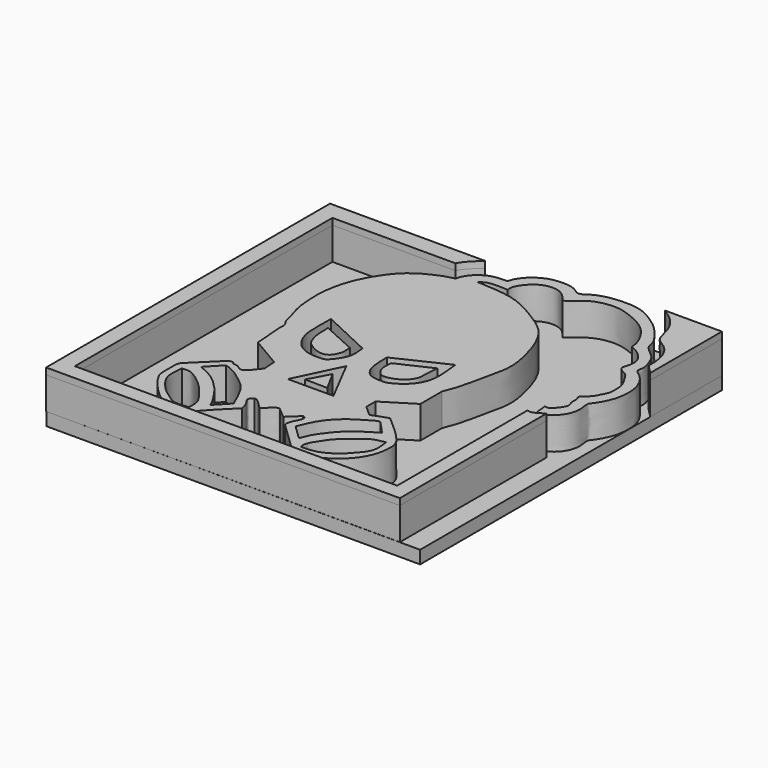
from build123d import *

# Parameters (mm, degrees)
F1_DEPTH = 5
F2_DEPTH = 1
F4_DEPTH = 2


# Not quite as in the source:
# - a feature names something its author has since deleted; it is built from what else it names


with BuildPart() as f1:
    # F0 (on Top) → F1 (new body)
    with BuildSketch(Plane.XY):
        with BuildLine():
            add(Edge.make_bspline(
                [(51.4540672302, 60.837585479), (51.9638869737, 60.5286784114), (53.1057350795, 59.8368163278), (54.9989821715, 57.6432839724), (55.3530510623, 54.4029967917), (56.8689093893, 53.8008966691), (58.5125441808, 52.2408419295), (59.0050335955, 49.7109659804), (58.9545683424, 48.7642556957), (58.9334107935, 48.3673475683)],
                knots=[0, 0, 0, 0, 0.1341689236, 0.3004994084, 0.4702111044, 0.5875997416, 0.7323290574, 0.8877790024, 1, 1, 1, 1], degree=3))
            add(Edge.make_bspline(
                [(58.9334107935, 48.3673475683), (59.3921567003, 47.8968396783), (59.850902607, 47.4263317883), (60.3096485138, 46.9558238983)],
                knots=[0, 0, 0, 0, 1.9714028846, 1.9714028846, 1.9714028846, 1.9714028846], degree=3))
            add(Edge.make_bspline(
                [(60.3096485138, 46.9558238983), (60.3096485138, 51.5830777586), (60.3096485138, 56.2103316188), (60.3096485138, 60.837585479)],
                knots=[0, 0, 0, 0, 13.8817615807, 13.8817615807, 13.8817615807, 13.8817615807], degree=3))
            add(Edge.make_bspline(
                [(60.3096485138, 60.837585479), (57.3577880859, 60.837585479), (54.4059276581, 60.837585479), (51.4540672302, 60.837585479)],
                knots=[0, 0, 0, 0, 8.8555812836, 8.8555812836, 8.8555812836, 8.8555812836], degree=3))
        make_face()
    extrude(amount=F1_DEPTH)


with BuildPart() as f1b:
    # F0 (on Top) → F1, piece 2 (new body)
    with BuildSketch(Plane.XY):
        with BuildLine():
            add(Edge.make_bspline(
                [(4.8520560376, 4.860504996), (21.518412667, 4.8331838722), (38.1847692964, 4.8058627484), (54.8511259258, 4.7785416245)],
                knots=[0, 0, 0, 0, 49.9991370693, 49.9991370693, 49.9991370693, 49.9991370693], degree=3))
            add(Edge.make_bspline(
                [(4.9181785434, 54.6599179506), (4.8961377082, 38.0601136324), (4.8740968729, 21.4603093142), (4.8520560376, 4.860504996)],
                knots=[0, 0, 0, 0, 49.7994568525, 49.7994568525, 49.7994568525, 49.7994568525], degree=3))
            add(Edge.make_bspline(
                [(23.9754598588, 54.6599179506), (17.6230327537, 54.6599179506), (11.2706056486, 54.6599179506), (4.9181785434, 54.6599179506)],
                knots=[0, 0, 0, 0, 19.0572813153, 19.0572813153, 19.0572813153, 19.0572813153], degree=3))
            add(Edge.make_bspline(
                [(26.3510439545, 57.3983192444), (25.3768845665, 56.4834475414), (24.4027251785, 55.5685758385), (23.9754598588, 54.6599179506)],
                knots=[0, 0, 0, 0, 0.5683118299, 0.5683118299, 0.5683118299, 0.5683118299], degree=3))
            add(Edge.make_bspline(
                [(2.3493634071, 57.3983192444), (10.5748367496, 57.3983192444), (18.125570612, 57.3983192444), (26.3510439545, 57.3983192444)],
                knots=[0, 0, 0, 0, 24.0016805474, 24.0016805474, 24.0016805474, 24.0016805474], degree=3))
            add(Edge.make_bspline(
                [(2.3493634071, 2.4174780119), (2.3493634071, 20.7312301112), (2.3493634071, 39.0845671451), (2.3493634071, 57.3983192444)],
                knots=[0, 0, 0, 0, 54.9808412325, 54.9808412325, 54.9808412325, 54.9808412325], degree=3))
            add(Edge.make_bspline(
                [(57.154417038, 2.4174780119), (38.8860658277, 2.4174780119), (20.6177146174, 2.4174780119), (2.3493634071, 2.4174780119)],
                knots=[0, 0, 0, 0, 54.8050536308, 54.8050536308, 54.8050536308, 54.8050536308], degree=3))
            add(Edge.make_bspline(
                [(57.154417038, 30.8391451836), (57.154417038, 21.3652561263), (57.154417038, 11.8913670691), (57.154417038, 2.4174780119)],
                knots=[0, 0, 0, 0, 28.4216671716, 28.4216671716, 28.4216671716, 28.4216671716], degree=3))
            add(Edge.make_bspline(
                [(56.1751872301, 30.2456729114), (56.3446747926, 30.3468590463), (56.7052673113, 30.5024971432), (57.0361231665, 30.7883044027), (57.154417038, 30.8391451836)],
                knots=[0.4614999783, 0.4614999783, 0.4614999783, 0.4614999783, 0.6787072438, 0.881944889, 0.881944889, 0.881944889, 0.881944889], degree=3))
            add(Edge.make_bspline(
                [(54.8511259258, 29.9786105752), (55.1455810804, 29.9474229205), (55.6857627215, 29.8902087804), (56.0113746232, 30.147874794), (56.1751872301, 30.2456729114)],
                knots=[0, 0, 0, 0, 0.2515654682, 0.4614999783, 0.4614999783, 0.4614999783, 0.4614999783], degree=3))
            add(Edge.make_bspline(
                [(54.8511259258, 29.7412201762), (54.8511259258, 29.8203503092), (54.8511259258, 29.8994804422), (54.8511259258, 29.9786105752)],
                knots=[0, 0, 0, 0, 0.237390399, 0.237390399, 0.237390399, 0.237390399], degree=3))
            add(Edge.make_bspline(
                [(54.8511259258, 4.7785416245), (54.8511259258, 13.0994344751), (54.8511259258, 21.4203273257), (54.8511259258, 29.7412201762)],
                knots=[0, 0, 0, 0, 24.9626785517, 24.9626785517, 24.9626785517, 24.9626785517], degree=3))
        make_face()
    extrude(amount=F1_DEPTH)


with BuildPart() as f1c:
    # F0 (on Top) → F1, piece 3 (new body)
    with BuildSketch(Plane.XY):
        with BuildLine():
            add(Edge.make_bspline(
                [(23.6329138279, 52.5964461267), (24.1818682601, 52.7461618185), (24.7308226923, 52.8958775103), (25.2797771245, 53.0455932021)],
                knots=[0, 0, 0, 0, 1.7070125404, 1.7070125404, 1.7070125404, 1.7070125404], degree=3))
            add(Edge.make_bspline(
                [(16.6953094304, 29.7442097217), (16.7411494158, 30.0597253678), (16.8346932753, 30.703585765), (16.1172664025, 31.527469058), (15.9920702036, 32.4892911415), (15.5262018988, 33.9022358039), (14.9877927895, 35.7559845442), (14.8019028777, 39.1876871759), (14.9425896683, 41.0184854519), (15.5349488179, 44.2279557805), (17.7090883866, 48.4871885716), (20.3947770421, 51.2022443546), (22.5699612299, 52.1387846708), (23.6329138279, 52.5964461267)],
                knots=[0, 0, 0, 0, 0.0581906098, 0.1187472939, 0.1778066529, 0.2499088208, 0.3358728435, 0.446880626, 0.5297458769, 0.6369929361, 0.7699468037, 0.8875793397, 1, 1, 1, 1], degree=3))
            add(Edge.make_bspline(
                [(16.6953094304, 29.7442097217), (16.8189499527, 28.1764511019), (16.9425904751, 26.6086924821), (17.0662309974, 25.0409338623)],
                knots=[0, 0, 0, 0, 4.717879462, 4.717879462, 4.717879462, 4.717879462], degree=3))
            add(Edge.make_bspline(
                [(17.0662309974, 25.0409338623), (18.6460409313, 24.1130304833), (20.2258508652, 23.1851271043), (21.8056607991, 22.2572237253)],
                knots=[0, 0, 0, 0, 5.4964749587, 5.4964749587, 5.4964749587, 5.4964749587], degree=3))
            add(Edge.make_bspline(
                [(21.8056607991, 22.2572237253), (21.8539827814, 21.5794897328), (21.9023047636, 20.9017557402), (21.9506267458, 20.2240217477)],
                knots=[0, 0, 0, 0, 2.038363414, 2.038363414, 2.038363414, 2.038363414], degree=3))
            add(Edge.make_bspline(
                [(21.9506267458, 20.2240217477), (21.333399398, 19.3876620701), (20.4237705446, 18.1550904784), (19.6675991421, 18.2369442462), (19.4042310191, 18.4234991753), (19.2801747471, 18.5113735497)],
                knots=[0, 0, 0, 0, 0.5275400347, 0.7774536215, 1, 1, 1, 1], degree=3))
            add(Edge.make_bspline(
                [(19.2801747471, 18.5113735497), (19.1605442292, 18.6046064616), (18.8964371747, 18.8104357949), (17.9988606757, 18.7690618062), (18.1630105259, 19.1715563199), (17.668384742, 19.1271965384), (17.3401199281, 19.0977565944)],
                knots=[0, 0, 0, 0, 0.2492135644, 0.5501862029, 0.7014752421, 1, 1, 1, 1], degree=3))
            add(Edge.make_bspline(
                [(17.3401199281, 19.0977565944), (15.9746278077, 17.7570494513), (14.6091356874, 16.4163423081), (13.243643567, 15.075635165)],
                knots=[0, 0, 0, 0, 5.7409563115, 5.7409563115, 5.7409563115, 5.7409563115], degree=3))
            add(Edge.make_bspline(
                [(13.243643567, 15.075635165), (13.1469812007, 14.9553622576), (12.8876584706, 14.6326979166), (12.9091331187, 13.2140349724), (12.8972099147, 11.3443591214), (13.2141228559, 10.5927181519), (13.8701516993, 9.5220356732), (14.6843078227, 8.5775849916), (15.9371129223, 7.1787648885), (17.6735731076, 5.853426051), (19.2182216843, 5.4657589264), (21.5649034696, 5.1720993414), (22.7222815558, 6.7413725499), (24.5478775436, 8.632399002), (25.7528635399, 9.8050942862), (26.3491775841, 10.3854285553)],
                knots=[0, 0, 0, 0, 0.0427668755, 0.1147336171, 0.1978923302, 0.252417499, 0.3184312013, 0.3865475344, 0.4698565501, 0.5583403323, 0.6360042741, 0.7240610103, 0.805005513, 0.9035026536, 1, 1, 1, 1], degree=3))
            add(Edge.make_bspline(
                [(26.3491775841, 10.3854285553), (26.3085010545, 10.5626896394), (26.2157529789, 10.9668692632), (25.9082855772, 11.8069959782), (25.1293913766, 12.7618461983), (25.6672707359, 13.1498958646), (25.9190015495, 13.33150547)],
                knots=[0, 0, 0, 0, 0.2084750741, 0.4753518091, 0.7544614537, 1, 1, 1, 1], degree=3))
            add(Edge.make_bspline(
                [(25.9190015495, 13.33150547), (25.9934808152, 13.3533379237), (26.2855093706, 13.4389416129), (27.1795420123, 12.5176051233), (27.8455596417, 11.8312472478)],
                knots=[0, 0, 0, 0, 0.2550410373, 1, 1, 1, 1], degree=3))
            add(Edge.make_bspline(
                [(27.8455596417, 11.8312472478), (27.8841573745, 11.803066358), (27.9227551073, 11.7748854682), (27.9613528401, 11.7467045784)],
                knots=[0, 0, 0, 0, 0.1433719907, 0.1433719907, 0.1433719907, 0.1433719907], degree=3))
            add(Edge.make_bspline(
                [(27.9613528401, 11.7467045784), (28.6060407165, 12.3853184901), (29.5122160489, 13.2829562382), (29.8725511163, 13.1726508141), (29.9765300006, 13.1408208981)],
                knots=[0, 0, 0, 0, 0.7114383425, 1, 1, 1, 1], degree=3))
            add(Edge.make_bspline(
                [(29.9765300006, 13.1408208981), (30.5281480153, 12.6761154582), (31.0797660301, 12.2114100183), (31.6313840449, 11.7467045784)],
                knots=[0, 0, 0, 0, 2.1638165867, 2.1638165867, 2.1638165867, 2.1638165867], degree=3))
            add(Edge.make_bspline(
                [(31.6313840449, 11.7467045784), (32.216536502, 12.3016138872), (32.8016889592, 12.8565231959), (33.3868414164, 13.4114325047)],
                knots=[0, 0, 0, 0, 2.419287013, 2.419287013, 2.419287013, 2.419287013], degree=3))
            add(Edge.make_bspline(
                [(33.3868414164, 13.4114325047), (33.5486950986, 13.3552916908), (33.8867448156, 13.238035253), (33.8179715888, 12.567413562), (33.4850854432, 12.015322984), (33.0332814649, 11.0514679637), (33.0377002003, 10.5395339776), (33.0397188663, 10.3056607768)],
                knots=[0, 0, 0, 0, 0.1650161295, 0.3446548457, 0.5448874038, 0.7920852248, 1, 1, 1, 1], degree=3))
            add(Edge.make_bspline(
                [(33.0397188663, 10.3056607768), (34.6381564935, 8.7701914211), (36.2365941207, 7.2347220654), (37.8350317478, 5.6992527097)],
                knots=[0, 0, 0, 0, 6.649362444, 6.649362444, 6.649362444, 6.649362444], degree=3))
            add(Edge.make_bspline(
                [(37.8350317478, 5.6992527097), (38.2359105795, 5.6037565979), (39.1362241923, 5.3919598538), (41.3365022802, 5.5014322365), (42.590198239, 6.7142053907), (44.6345343863, 7.9569178764), (46.4813202402, 10.6288684465), (46.8725075082, 13.4278642872), (46.6458193339, 15.4761556325), (43.7917175879, 17.9417535437), (41.9382452965, 19.5452924818)],
                knots=[0, 0, 0, 0, 0.0908879872, 0.2042224773, 0.3063473936, 0.4269823327, 0.5683083629, 0.6977953089, 0.8037676819, 1, 1, 1, 1], degree=3))
            add(Edge.make_bspline(
                [(41.9382452965, 19.5452924818), (41.7742155002, 19.4995135268), (41.3754645957, 19.3882264306), (40.2849393648, 18.9547964214), (39.7226906231, 18.7309311117), (39.4596159458, 18.6261851341)],
                knots=[0, 0, 0, 0, 0.2710565406, 0.6589293117, 1, 1, 1, 1], degree=3))
            add(Edge.make_bspline(
                [(39.4596159458, 18.6261851341), (38.9180878798, 19.1119220108), (38.3765598138, 19.5976588875), (37.8350317478, 20.0833957642)],
                knots=[0, 0, 0, 0, 2.1823695006, 2.1823695006, 2.1823695006, 2.1823695006], degree=3))
            add(Edge.make_bspline(
                [(37.8350317478, 20.0833957642), (37.8350317478, 20.6729732454), (37.8350317478, 21.2625507265), (37.8350317478, 21.8521282077)],
                knots=[0, 0, 0, 0, 1.7687324435, 1.7687324435, 1.7687324435, 1.7687324435], degree=3))
            add(Edge.make_bspline(
                [(37.8350317478, 21.8521282077), (39.381377399, 22.8159365555), (40.9277230501, 23.7797449032), (42.4740687013, 24.743553251)],
                knots=[0, 0, 0, 0, 5.4663518581, 5.4663518581, 5.4663518581, 5.4663518581], degree=3))
            add(Edge.make_bspline(
                [(42.4740687013, 24.743553251), (42.4740687013, 26.1413361877), (42.4740687013, 27.5391191244), (42.4740687013, 28.9369020611)],
                knots=[0, 0, 0, 0, 4.1933488101, 4.1933488101, 4.1933488101, 4.1933488101], degree=3))
            add(Edge.make_bspline(
                [(42.4740687013, 28.9369020611), (42.7782509399, 29.6896295627), (43.4615747648, 31.3805785076), (44.179786716, 35.3676298617), (45.1619240466, 38.8944675844), (44.3939051333, 43.1779076385), (42.4534637338, 48.7027158005), (37.8233233172, 51.4880268363), (34.0302323882, 53.6455249326), (30.3441072705, 53.8718574183), (28.4098464997, 53.9662561815)],
                knots=[0, 0, 0, 0, 0.0959239421, 0.2154863325, 0.3290047924, 0.4521753396, 0.594301552, 0.7299651508, 0.8549820054, 0.9896016982, 0.9896016982, 0.9896016982, 0.9896016982], degree=3))
            add(Edge.make_bspline(
                [(28.4098464997, 53.9662561815), (28.2604402213, 53.973547736), (28.1108965307, 53.9807023452), (27.9613528401, 53.9878569543)],
                knots=[0.9896016982, 0.9896016982, 0.9896016982, 0.9896016982, 1, 1, 1, 1], degree=3))
            add(Edge.make_bspline(
                [(27.9613528401, 53.9878569543), (28.2577815438, 54.2322938946), (29.0197904968, 54.8606511845), (30.8986250138, 54.75163223), (32.0465750992, 54.685022682)],
                knots=[0, 0, 0, 0, 0.3890094763, 1, 1, 1, 1], degree=3))
            add(Edge.make_bspline(
                [(32.0465750992, 54.685022682), (32.0030570843, 54.9603139422), (31.8960262096, 55.6373821501), (33.0058570002, 57.3043329036), (34.6608708244, 58.5585145213), (37.3761968026, 58.6343066487), (38.4691053223, 57.2842579703), (39.0217341483, 56.6016063094)],
                knots=[0, 0, 0, 0, 0.1364189236, 0.3355170669, 0.5454458617, 0.7701548526, 1, 1, 1, 1], degree=3))
            add(Edge.make_bspline(
                [(39.0217341483, 56.6016063094), (39.3457847148, 56.852344862), (40.0565789865, 57.4023316397), (41.4546178184, 58.6184143391), (43.4851207218, 59.2978722978), (45.5225485064, 59.3662645176), (47.2365071434, 58.8924142967), (49.7756335287, 57.8331653424), (51.6817843812, 56.247162881), (53.0214598266, 53.6881433446), (53.0581333298, 52.7902749209), (53.0726537108, 52.4347759783)],
                knots=[0, 0, 0, 0, 0.0893545777, 0.1959963308, 0.3112705226, 0.4221335419, 0.5272131137, 0.6562268996, 0.7826342982, 0.9139369699, 1, 1, 1, 1], degree=3))
            add(Edge.make_bspline(
                [(53.0726537108, 52.4347759783), (53.3844845117, 52.3108211533), (54.1252668721, 52.01635522), (55.5754253441, 50.766966304), (56.0672880612, 49.3942507672), (55.7217534832, 47.9682197362), (55.4931357773, 47.4938705794), (55.8111531414, 46.8224962583), (56.9823574012, 46.4525364988), (57.4686896746, 45.5578943128), (57.9620984754, 44.8063345229), (58.5209609315, 43.7886786016), (58.547767924, 42.7111266891), (58.6090971939, 41.4291363456), (57.988064782, 40.3079990255), (57.5090190758, 39.1813677792), (55.9516965504, 38.1636576583), (56.5919912725, 37.7404775491), (56.3250122319, 36.4575018693), (56.9647449517, 35.6953071099), (56.1161024627, 34.3499216103), (55.2500631112, 33.4513027359), (54.5236237133, 33.7303949316), (54.7500839578, 33.1407038806), (54.7113907814, 32.2726423357), (54.8413917652, 31.8719840609)],
                knots=[0, 0, 0, 0, 0.0448396862, 0.1027973287, 0.1540382314, 0.2041526429, 0.2339315331, 0.2672558728, 0.3133640521, 0.3554264447, 0.3960040548, 0.4410187638, 0.4851897275, 0.5327623965, 0.5798295918, 0.6289543934, 0.6812242363, 0.7098825078, 0.7563225861, 0.7959410868, 0.8473453234, 0.8943816793, 0.9237098639, 0.9505994993, 1, 1, 1, 1], degree=3))
            add(Edge.make_bspline(
                [(50.2767972648, 59.3599267304), (50.6166012713, 59.1406105779), (51.315587007, 58.6894715118), (52.3421445307, 57.7425080218), (53.4185302986, 56.426271044), (54.6045883457, 54.7487703423), (54.4657630765, 53.5424084336), (56.3794303899, 52.1470924237), (56.9528348366, 51.3589002503), (57.5431847997, 49.7983121362), (57.7258520997, 48.7992372882), (57.3071433348, 47.8799260339), (58.6990952057, 47.0870823951), (59.7141760403, 45.6316290257), (60.256477453, 44.1395211131), (60.3225445964, 42.3493394989), (60.0711832054, 40.3295292003), (58.8102474072, 38.011920833), (58.1138617589, 37.4308333829), (58.6090848995, 35.6802681712), (58.0779514482, 33.5855164482), (56.4751219569, 32.0159222836), (55.3264026447, 31.8433918777), (54.8413917652, 31.8719840609)],
                knots=[0, 0, 0, 0, 0.0356592621, 0.0733616155, 0.1163119468, 0.1614301837, 0.1954735807, 0.2428003716, 0.2761343564, 0.3169772532, 0.3497227063, 0.3781574066, 0.4160031284, 0.4594766221, 0.4997977615, 0.5421432001, 0.5892397134, 0.6407735561, 0.6694750292, 0.7102701616, 0.7577630881, 0.8062100078, 0.8398516659, 0.8398516659, 0.8398516659, 0.8398516659], degree=3))
            add(Edge.make_bspline(
                [(38.9672592282, 59.3599267304), (39.608079645, 59.1738823301), (40.1305635938, 59.6805706538), (41.4375664612, 60.4109334097), (43.3072109154, 60.8771613655), (45.6142336602, 61.0176578595), (47.9512009953, 60.7776391576), (49.5092640164, 59.9002861195), (50.2767972648, 59.3599267304)],
                knots=[0, 0, 0, 0, 0.1335248261, 0.2751443287, 0.4408792293, 0.6223616297, 0.8037992646, 1, 1, 1, 1], degree=3))
            add(Edge.make_bspline(
                [(30.5821765214, 56.439127773), (30.6819426689, 56.7573363815), (30.8951705359, 57.4361157166), (31.8155627946, 58.6536909912), (32.9499524699, 59.5094168867), (34.5767150364, 60.3010181202), (37.6303922327, 60.3482327023), (38.4718062531, 59.6959897964), (38.9672592282, 59.3599267304)],
                knots=[0, 0, 0, 0, 0.1310135954, 0.2884008309, 0.4409120291, 0.6153010996, 0.8343745605, 1, 1, 1, 1], degree=3))
            add(Edge.make_bspline(
                [(25.2797771245, 53.0455932021), (25.3131320538, 53.2115700955), (25.382259253, 53.5555527699), (25.6499960752, 54.0885350469), (25.9723783787, 54.631855017), (26.4677703504, 55.1902173867), (27.5596415134, 56.0148849833), (28.8353856883, 56.4128910098), (29.974461845, 56.4299999108), (30.5821765214, 56.439127773)],
                knots=[0, 0, 0, 0, 0.1059960546, 0.2196739896, 0.3356921752, 0.4629857686, 0.633605129, 0.8045226922, 1, 1, 1, 1], degree=3))
        make_face()
        with BuildLine():
            add(Edge.make_bspline(
                [(14.1202360392, 13.9799248427), (14.534522447, 14.0221604457), (15.3762304164, 14.107970752), (16.5458010718, 13.4139388553), (17.9594208708, 12.3621955313), (19.4240247165, 10.8027768278), (20.9291595401, 8.7649974123), (21.1712321927, 7.8657743266), (21.141143953, 7.0463174558), (21.1249291897, 6.6047064029)],
                knots=[0, 0, 0, 0, 0.1269040312, 0.2578316169, 0.4092814242, 0.5821497101, 0.7628156944, 0.8721797148, 1, 1, 1, 1], degree=3))
            add(Edge.make_bspline(
                [(21.1249291897, 6.6047064029), (20.3348346944, 6.49656113), (18.8975632142, 6.2998326154), (17.6525381576, 7.2606785374), (16.1717948229, 8.2444174922), (14.9293990713, 9.6804335), (13.8489202224, 11.3409464244), (14.0249690411, 13.0533015635), (14.1202360392, 13.9799248427)],
                knots=[0, 0, 0, 0, 0.1765162855, 0.3211031395, 0.4795782903, 0.6437231916, 0.8072044887, 1, 1, 1, 1], degree=3))
        make_face(mode=Mode.SUBTRACT)
        with BuildLine():
            add(Edge.make_bspline(
                [(20.3866381198, 12.4512678012), (20.0754552605, 12.7859513335), (19.4414510073, 13.46783588), (18.3284060287, 14.4449773275), (16.9534484856, 15.2377783132), (16.0917135457, 15.5714541011), (15.6767740846, 15.7321244478)],
                knots=[0, 0, 0, 0, 0.2437976675, 0.4967135993, 0.7576593704, 1, 1, 1, 1], degree=3))
            add(Edge.make_bspline(
                [(15.6767740846, 15.7321244478), (16.375956436, 16.4739334335), (17.0751387874, 17.2157424192), (17.7743211389, 17.9575514048)],
                knots=[0, 0, 0, 0, 3.058141394, 3.058141394, 3.058141394, 3.058141394], degree=3))
            add(Edge.make_bspline(
                [(17.7743211389, 17.9575514048), (18.0497333451, 17.8835404898), (18.6658398296, 17.7179755524), (19.9116330348, 17.0359787254), (21.0156331317, 16.1718165788), (22.5735913543, 15.0081073708), (23.6956842391, 13.2040958117), (24.3956650949, 11.5808570102), (24.7683897614, 10.7165174559)],
                knots=[0, 0, 0, 0, 0.1218974367, 0.272688717, 0.4260658247, 0.6020650871, 0.7881082654, 1, 1, 1, 1], degree=3))
            add(Edge.make_bspline(
                [(24.7683897614, 10.7165174559), (24.1117688517, 10.0296664362), (23.4551479419, 9.3428154166), (22.7985270321, 8.6559643969)],
                knots=[0, 0, 0, 0, 2.8506557283, 2.8506557283, 2.8506557283, 2.8506557283], degree=3))
            add(Edge.make_bspline(
                [(22.7985270321, 8.6559643969), (22.6882949604, 8.9350561669), (22.4091990701, 9.6821060877), (20.8153935358, 11.9875680537), (20.3866381198, 12.4512678012)],
                knots=[0, 0, 0, 0, 0.3702373056, 1, 1, 1, 1], degree=3))
        make_face(mode=Mode.SUBTRACT)
        with BuildLine():
            add(Edge.make_bspline(
                [(38.2436583284, 8.0758738545), (38.282603656, 8.2085083864), (38.3872227162, 8.5644506951), (39.246454388, 9.7347849235), (39.5328454287, 10.3637737491), (40.839289552, 11.7965820716), (42.1614963079, 12.6176050451), (43.66240807, 14.1359064033), (44.9059359667, 14.1199337936), (45.5148816109, 14.3478652462)],
                knots=[0, 0, 0, 0, 0.0863418612, 0.2308009263, 0.3382328579, 0.5030926119, 0.6615772328, 0.8339851684, 1, 1, 1, 1], degree=3))
            add(Edge.make_bspline(
                [(45.5148816109, 14.3478652462), (45.6420752419, 13.4791301927), (45.8913585121, 11.775743474), (44.5059630164, 10.027013908), (43.1083449002, 8.5330827774), (42.0787290132, 7.8918694542), (41.4013525263, 7.4817547716), (40.2815787825, 7.0394763881), (38.9062756036, 6.9241477113), (38.2436583284, 6.9237181462)],
                knots=[0, 0, 0, 0, 0.1767542423, 0.3398403493, 0.5005380705, 0.6213994001, 0.7182177662, 0.8394731022, 1, 1, 1, 1], degree=3))
            add(Edge.make_bspline(
                [(38.2436583284, 6.9237181462), (38.0413430685, 7.2606434961), (38.0355916968, 7.7236100146), (38.2436583284, 8.0758738545)],
                knots=[0, 0, 0, 0, 1.1521557083, 1.1521557083, 1.1521557083, 1.1521557083], degree=3))
        make_face(mode=Mode.SUBTRACT)
        with BuildLine():
            add(Edge.make_bspline(
                [(34.356020391, 10.7165174559), (35.1072673996, 9.9950001265), (35.8585144083, 9.273482797), (36.6097614169, 8.5519654676)],
                knots=[0, 0, 0, 0, 3.1248414235, 3.1248414235, 3.1248414235, 3.1248414235], degree=3))
            add(Edge.make_bspline(
                [(41.6493713856, 18.030108884), (41.53428509, 18.0481312377), (41.2166889903, 18.0978663449), (40.1652640782, 17.3971102257), (38.02250188, 16.2595965366), (36.1177488176, 14.3202485646), (35.0499709055, 12.4945241032), (34.5831036608, 11.298339293), (34.356020391, 10.7165174559)],
                knots=[0, 0, 0, 0, 0.0790539848, 0.2181600956, 0.4222923482, 0.6358267843, 0.8228668952, 1, 1, 1, 1], degree=3))
            add(Edge.make_bspline(
                [(43.5736142099, 15.9420669079), (42.9321999351, 16.6380808999), (42.2907856603, 17.3340948919), (41.6493713856, 18.030108884)],
                knots=[0, 0, 0, 0, 2.8394770189, 2.8394770189, 2.8394770189, 2.8394770189], degree=3))
            add(Edge.make_bspline(
                [(36.6097614169, 8.5519654676), (36.7609252633, 8.9580807925), (37.076846154, 9.8068307961), (37.8540365506, 11.165293063), (40.0915780551, 13.9247570133), (42.3793308345, 15.2501614931), (43.5736142099, 15.9420669079)],
                knots=[0, 0, 0, 0, 0.1815202157, 0.3793633835, 0.6760069533, 1, 1, 1, 1], degree=3))
        make_face(mode=Mode.SUBTRACT)
        with BuildLine():
            add(Edge.make_bspline(
                [(18.2253848761, 25.9095039219), (19.7932012379, 24.8927244296), (21.3610175997, 23.8759449373), (22.9288339615, 22.859165445)],
                knots=[0, 0, 0, 0, 5.6059787836, 5.6059787836, 5.6059787836, 5.6059787836], degree=3))
            add(Edge.make_bspline(
                [(35.1268388331, 51.6205057502), (34.9373060761, 51.6859761808), (34.4435343208, 51.8565400979), (32.7463134036, 52.5317364005), (31.1540028799, 52.7775351746), (29.20226834, 52.9999686325), (27.39503116, 52.6199878707), (25.2395596297, 51.8523533881), (23.6768101447, 51.4308467616), (21.905741835, 50.3006759854), (20.2978956546, 49.3784316912), (18.8565086268, 47.6361287327), (18.131289098, 46.136257308), (17.22396439, 44.3779957313), (16.4979240123, 41.8662009096), (16.1280611237, 40.6919669371), (16.0427080812, 36.7833408989), (16.7348591622, 35.1526023242), (17.1587506324, 33.364694616), (17.681976015, 31.4819251063), (17.9251427726, 30.0434288752), (18.1403398876, 26.691035276), (18.2046078573, 26.1004368852), (18.2253848761, 25.9095039219)],
                knots=[0, 0, 0, 0, 0.02900212, 0.0755564785, 0.1208844055, 0.1688769903, 0.2166399622, 0.2689181228, 0.313632777, 0.3632839387, 0.4113560285, 0.4628969995, 0.5077167586, 0.5573486541, 0.6124219379, 0.6530438275, 0.7203467867, 0.7678830276, 0.8144967259, 0.862159853, 0.9065259076, 0.9697810124, 1, 1, 1, 1], degree=3))
            add(Edge.make_bspline(
                [(41.3381122053, 25.9095039219), (41.2528435968, 27.0578702938), (41.0964559216, 29.163732736), (42.1377728682, 31.2490887542), (42.3744237568, 33.8625011917), (43.4348721882, 36.6242029024), (43.471011644, 41.9919572305), (41.7916098691, 46.9294993676), (37.9280368649, 50.0634025354), (36.0521089705, 51.2426520868), (35.1268388331, 51.6205057502)],
                knots=[0, 0, 0, 0, 0.1188752723, 0.2180780383, 0.3224001799, 0.4356816344, 0.587165154, 0.7379272082, 0.8826623647, 1, 1, 1, 1], degree=3))
            add(Edge.make_bspline(
                [(36.526337266, 22.859165445), (38.1302622457, 23.8759449373), (39.7341872255, 24.8927244296), (41.3381122053, 25.9095039219)],
                knots=[0, 0, 0, 0, 5.6971697263, 5.6971697263, 5.6971697263, 5.6971697263], degree=3))
            add(Edge.make_bspline(
                [(36.526337266, 19.5542983711), (36.526337266, 20.655920729), (36.526337266, 21.757543087), (36.526337266, 22.859165445)],
                knots=[0, 0, 0, 0, 3.3048670739, 3.3048670739, 3.3048670739, 3.3048670739], degree=3))
            add(Edge.make_bspline(
                [(38.2046811283, 17.9180298001), (37.6452331742, 18.4634526571), (37.0857852201, 19.0088755141), (36.526337266, 19.5542983711)],
                knots=[0, 0, 0, 0, 2.3439737534, 2.3439737534, 2.3439737534, 2.3439737534], degree=3))
            add(Edge.make_bspline(
                [(34.6129946411, 13.9643186703), (34.5816127649, 14.1002101875), (34.4950581047, 14.4750139123), (35.5055036707, 15.6010084977), (36.2346318108, 16.5251335261), (37.4807486317, 17.4061832853), (38.2046811283, 17.9180298001)],
                knots=[0, 0, 0, 0, 0.1483897971, 0.4092753529, 0.6568180756, 1, 1, 1, 1], degree=3))
            add(Edge.make_bspline(
                [(33.4442332387, 14.9165205657), (33.8338203728, 14.5991199339), (34.2234075069, 14.2817193021), (34.6129946411, 13.9643186703)],
                knots=[0, 0, 0, 0, 1.5075449132, 1.5075449132, 1.5075449132, 1.5075449132], degree=3))
            add(Edge.make_bspline(
                [(31.6093377769, 13.1870433688), (32.2209695975, 13.7635357678), (32.8326014181, 14.3400281668), (33.4442332387, 14.9165205657)],
                knots=[0, 0, 0, 0, 2.5214941464, 2.5214941464, 2.5214941464, 2.5214941464], degree=3))
            add(Edge.make_bspline(
                [(29.7852475196, 14.9165205657), (30.3932776054, 14.3400281668), (31.0013076911, 13.7635357678), (31.6093377769, 13.1870433688)],
                knots=[0, 0, 0, 0, 2.5136421069, 2.5136421069, 2.5136421069, 2.5136421069], degree=3))
            add(Edge.make_bspline(
                [(27.9327519238, 13.1870433688), (28.5502504557, 13.7635357678), (29.1677489877, 14.3400281668), (29.7852475196, 14.9165205657)],
                knots=[0, 0, 0, 0, 2.5343305442, 2.5343305442, 2.5343305442, 2.5343305442], degree=3))
            add(Edge.make_bspline(
                [(21.1888644844, 17.9180298001), (21.6501197547, 17.6493894859), (22.5523660575, 17.1239109802), (23.4783273977, 16.0462125164), (24.4417054378, 14.9229631595), (24.7215230191, 13.9932503776), (25.1802507625, 13.8590779457), (25.4944401106, 14.5026222276), (25.9381383376, 14.8053516141), (26.3960732883, 14.9078004005), (26.7625518508, 14.2037383036), (27.2285451576, 13.9187214483), (27.6763147927, 13.4534841879), (27.9327519238, 13.1870433688)],
                knots=[0, 0, 0, 0, 0.1259897337, 0.246444385, 0.3701306267, 0.4659318653, 0.521937027, 0.6024971332, 0.6774795547, 0.7388842262, 0.8227194123, 0.8984716208, 1, 1, 1, 1], degree=3))
            add(Edge.make_bspline(
                [(22.9288339615, 19.5542983711), (22.3488441358, 19.0088755141), (21.7688543101, 18.4634526571), (21.1888644844, 17.9180298001)],
                knots=[0, 0, 0, 0, 2.3884866794, 2.3884866794, 2.3884866794, 2.3884866794], degree=3))
            add(Edge.make_bspline(
                [(22.9288339615, 22.859165445), (22.9288339615, 21.757543087), (22.9288339615, 20.655920729), (22.9288339615, 19.5542983711)],
                knots=[0, 0, 0, 0, 3.3048670739, 3.3048670739, 3.3048670739, 3.3048670739], degree=3))
        make_face(mode=Mode.SUBTRACT)
        with BuildLine():
            add(Edge.make_bspline(
                [(35.1268388331, 51.6205057502), (34.9373060761, 51.6859761808), (34.4435343208, 51.8565400979), (32.7463134036, 52.5317364005), (31.1540028799, 52.7775351746), (29.20226834, 52.9999686325), (27.39503116, 52.6199878707), (25.2395596297, 51.8523533881), (23.6768101447, 51.4308467616), (21.905741835, 50.3006759854), (20.2978956546, 49.3784316912), (18.8565086268, 47.6361287327), (18.131289098, 46.136257308), (17.22396439, 44.3779957313), (16.4979240123, 41.8662009096), (16.1280611237, 40.6919669371), (16.0427080812, 36.7833408989), (16.7348591622, 35.1526023242), (17.1587506324, 33.364694616), (17.681976015, 31.4819251063), (17.9251427726, 30.0434288752), (18.1403398876, 26.691035276), (18.2046078573, 26.1004368852), (18.2253848761, 25.9095039219)],
                knots=[0, 0, 0, 0, 0.02900212, 0.0755564785, 0.1208844055, 0.1688769903, 0.2166399622, 0.2689181228, 0.313632777, 0.3632839387, 0.4113560285, 0.4628969995, 0.5077167586, 0.5573486541, 0.6124219379, 0.6530438275, 0.7203467867, 0.7678830276, 0.8144967259, 0.862159853, 0.9065259076, 0.9697810124, 1, 1, 1, 1], degree=3))
            add(Edge.make_bspline(
                [(18.2253848761, 25.9095039219), (19.7932012379, 24.8927244296), (21.3610175997, 23.8759449373), (22.9288339615, 22.859165445)],
                knots=[0, 0, 0, 0, 5.6059787836, 5.6059787836, 5.6059787836, 5.6059787836], degree=3))
            add(Edge.make_bspline(
                [(22.9288339615, 22.859165445), (22.9288339615, 21.757543087), (22.9288339615, 20.655920729), (22.9288339615, 19.5542983711)],
                knots=[0, 0, 0, 0, 3.3048670739, 3.3048670739, 3.3048670739, 3.3048670739], degree=3))
            add(Edge.make_bspline(
                [(22.9288339615, 19.5542983711), (22.3488441358, 19.0088755141), (21.7688543101, 18.4634526571), (21.1888644844, 17.9180298001)],
                knots=[0, 0, 0, 0, 2.3884866794, 2.3884866794, 2.3884866794, 2.3884866794], degree=3))
            add(Edge.make_bspline(
                [(21.1888644844, 17.9180298001), (21.6501197547, 17.6493894859), (22.5523660575, 17.1239109802), (23.4783273977, 16.0462125164), (24.4417054378, 14.9229631595), (24.7215230191, 13.9932503776), (25.1802507625, 13.8590779457), (25.4944401106, 14.5026222276), (25.9381383376, 14.8053516141), (26.3960732883, 14.9078004005), (26.7625518508, 14.2037383036), (27.2285451576, 13.9187214483), (27.6763147927, 13.4534841879), (27.9327519238, 13.1870433688)],
                knots=[0, 0, 0, 0, 0.1259897337, 0.246444385, 0.3701306267, 0.4659318653, 0.521937027, 0.6024971332, 0.6774795547, 0.7388842262, 0.8227194123, 0.8984716208, 1, 1, 1, 1], degree=3))
            add(Edge.make_bspline(
                [(27.9327519238, 13.1870433688), (28.5502504557, 13.7635357678), (29.1677489877, 14.3400281668), (29.7852475196, 14.9165205657)],
                knots=[0, 0, 0, 0, 2.5343305442, 2.5343305442, 2.5343305442, 2.5343305442], degree=3))
            add(Edge.make_bspline(
                [(29.7852475196, 14.9165205657), (30.3932776054, 14.3400281668), (31.0013076911, 13.7635357678), (31.6093377769, 13.1870433688)],
                knots=[0, 0, 0, 0, 2.5136421069, 2.5136421069, 2.5136421069, 2.5136421069], degree=3))
            add(Edge.make_bspline(
                [(31.6093377769, 13.1870433688), (32.2209695975, 13.7635357678), (32.8326014181, 14.3400281668), (33.4442332387, 14.9165205657)],
                knots=[0, 0, 0, 0, 2.5214941464, 2.5214941464, 2.5214941464, 2.5214941464], degree=3))
            add(Edge.make_bspline(
                [(33.4442332387, 14.9165205657), (33.8338203728, 14.5991199339), (34.2234075069, 14.2817193021), (34.6129946411, 13.9643186703)],
                knots=[0, 0, 0, 0, 1.5075449132, 1.5075449132, 1.5075449132, 1.5075449132], degree=3))
            add(Edge.make_bspline(
                [(34.6129946411, 13.9643186703), (34.5816127649, 14.1002101875), (34.4950581047, 14.4750139123), (35.5055036707, 15.6010084977), (36.2346318108, 16.5251335261), (37.4807486317, 17.4061832853), (38.2046811283, 17.9180298001)],
                knots=[0, 0, 0, 0, 0.1483897971, 0.4092753529, 0.6568180756, 1, 1, 1, 1], degree=3))
            add(Edge.make_bspline(
                [(38.2046811283, 17.9180298001), (37.6452331742, 18.4634526571), (37.0857852201, 19.0088755141), (36.526337266, 19.5542983711)],
                knots=[0, 0, 0, 0, 2.3439737534, 2.3439737534, 2.3439737534, 2.3439737534], degree=3))
            add(Edge.make_bspline(
                [(36.526337266, 19.5542983711), (36.526337266, 20.655920729), (36.526337266, 21.757543087), (36.526337266, 22.859165445)],
                knots=[0, 0, 0, 0, 3.3048670739, 3.3048670739, 3.3048670739, 3.3048670739], degree=3))
            add(Edge.make_bspline(
                [(36.526337266, 22.859165445), (38.1302622457, 23.8759449373), (39.7341872255, 24.8927244296), (41.3381122053, 25.9095039219)],
                knots=[0, 0, 0, 0, 5.6971697263, 5.6971697263, 5.6971697263, 5.6971697263], degree=3))
            add(Edge.make_bspline(
                [(41.3381122053, 25.9095039219), (41.2528435968, 27.0578702938), (41.0964559216, 29.163732736), (42.1377728682, 31.2490887542), (42.3744237568, 33.8625011917), (43.4348721882, 36.6242029024), (43.471011644, 41.9919572305), (41.7916098691, 46.9294993676), (37.9280368649, 50.0634025354), (36.0521089705, 51.2426520868), (35.1268388331, 51.6205057502)],
                knots=[0, 0, 0, 0, 0.1188752723, 0.2180780383, 0.3224001799, 0.4356816344, 0.587165154, 0.7379272082, 0.8826623647, 1, 1, 1, 1], degree=3))
        make_face()
        with BuildLine():
            add(Edge.make_bspline(
                [(25.8770771325, 19.8076292872), (28.2311228414, 19.8133333276), (30.5851685504, 19.8190373679), (32.9392142594, 19.8247414082)],
                knots=[0, 0, 0, 0, 7.0621578589, 7.0621578589, 7.0621578589, 7.0621578589], degree=3))
            add(Edge.make_bspline(
                [(29.2910933495, 26.8796570599), (28.1530879438, 24.522314469), (27.0150825381, 22.1649718781), (25.8770771325, 19.8076292872)],
                knots=[0, 0, 0, 0, 7.8529665444, 7.8529665444, 7.8529665444, 7.8529665444], degree=3))
            add(Edge.make_bspline(
                [(32.9392142594, 19.8247414082), (31.7231739561, 22.1763799588), (30.5071336528, 24.5280185093), (29.2910933495, 26.8796570599)],
                knots=[0, 0, 0, 0, 7.9423309567, 7.9423309567, 7.9423309567, 7.9423309567], degree=3))
        make_face(mode=Mode.SUBTRACT)
        with BuildLine():
            add(Edge.make_bspline(
                [(20.1291833073, 35.375803709), (22.7243347714, 34.1613193353), (25.3194862356, 32.9468349616), (27.9146376997, 31.7323505878)],
                knots=[0, 0, 0, 0, 8.5958158858, 8.5958158858, 8.5958158858, 8.5958158858], degree=3))
            add(Edge.make_bspline(
                [(27.9146376997, 31.7323505878), (28.0343551309, 30.8338881855), (28.2668458403, 29.0890782671), (26.6654163773, 27.0303377936), (26.0856876922, 26.5243961088), (23.7344430768, 26.4934649428), (21.5355687551, 27.4680460747), (20.2291694051, 29.9224536375), (20.0449831462, 32.0293156965), (20.0990227066, 34.1770876086), (20.1291833073, 35.375803709)],
                knots=[0, 0, 0, 0, 0.1366623345, 0.265397635, 0.3371644265, 0.4600439527, 0.5902231483, 0.724595357, 0.8462909502, 1, 1, 1, 1], degree=3))
        make_face(mode=Mode.SUBTRACT)
        with BuildLine():
            add(Edge.make_bspline(
                [(31.6983424127, 31.7323505878), (34.2605672777, 32.9468349616), (36.8227921426, 34.1613193353), (39.3850170076, 35.375803709)],
                knots=[0, 0, 0, 0, 8.5064514913, 8.5064514913, 8.5064514913, 8.5064514913], degree=3))
            add(Edge.make_bspline(
                [(39.3850170076, 35.375803709), (39.4940109088, 34.452209134), (39.7094439432, 32.6105381137), (39.6250930298, 29.8333252836), (37.9677937858, 27.6314010503), (35.9879574603, 26.5499126634), (35.3163498317, 26.4715402677), (33.2490634646, 26.4743703254), (32.2045963814, 27.6773984754), (31.7194736368, 29.1000180411), (31.7060660609, 30.7702066923), (31.6983424127, 31.7323505878)],
                knots=[0, 0, 0, 0, 0.1319407373, 0.2612152892, 0.3914545618, 0.5055186392, 0.5716514125, 0.6804936291, 0.7764773801, 0.871236873, 1, 1, 1, 1], degree=3))
        make_face(mode=Mode.SUBTRACT)
    extrude(amount=F1_DEPTH)


with BuildPart() as f1d:
    # F0 (on Top) → F1, piece 4 (new body)
    with BuildSketch(Plane.XY):
        with BuildLine():
            add(Edge.make_bspline(
                [(38.2763110101, 33.312600106), (36.5401804447, 32.5036222736), (34.8040498793, 31.6946444412), (33.0679193139, 30.8856666088)],
                knots=[0, 0, 0, 0, 5.7460725945, 5.7460725945, 5.7460725945, 5.7460725945], degree=3))
            add(Edge.make_bspline(
                [(33.0679193139, 30.8856666088), (32.9879255984, 30.2777483108), (32.8293638311, 29.0727461546), (34.0348899227, 27.3059171923), (36.0422532043, 27.8881974922), (37.271625218, 28.6554213976), (38.1428909751, 29.8993294408), (38.0700948109, 31.3198874981), (38.2032658577, 32.6067486904), (38.2763110101, 33.312600106)],
                knots=[0, 0, 0, 0, 0.1493855782, 0.2961087771, 0.4458049698, 0.5814103127, 0.7119506001, 0.8420031019, 1, 1, 1, 1], degree=3))
        make_face()
    extrude(amount=F1_DEPTH)


with BuildPart() as f1e:
    # F0 (on Top) → F1, piece 5 (new body)
    with BuildSketch(Plane.XY):
        with BuildLine():
            add(Edge.make_bspline(
                [(26.6392473131, 30.8856666088), (26.6715445648, 30.3299964852), (26.7246936664, 29.4155729263), (26.4346632619, 28.8332530849), (26.2064946439, 28.255132055), (25.730229935, 27.7905559705), (25.1061453756, 27.5714035594), (24.2439546506, 27.6836800217), (23.5058448629, 27.9779781634), (22.7391776668, 28.4216000866), (22.2099593794, 28.8528538512), (21.8035639666, 29.5031977717), (21.6955595993, 29.925651966), (21.6434840113, 30.1293432713)],
                knots=[0, 0, 0, 0, 0.1265956335, 0.2083286914, 0.2887657686, 0.3718442407, 0.4549403149, 0.5502997347, 0.6440360205, 0.7410388396, 0.8270921067, 0.9166304065, 1, 1, 1, 1], degree=3))
            add(Edge.make_bspline(
                [(26.6392473131, 30.8856666088), (24.8637584349, 31.6946444412), (23.0882695566, 32.5036222736), (21.3127806783, 33.312600106)],
                knots=[0, 0, 0, 0, 5.8533112861, 5.8533112861, 5.8533112861, 5.8533112861], degree=3))
            add(Edge.make_bspline(
                [(21.6434840113, 30.1293432713), (21.5933438985, 30.2969754753), (21.4889886408, 30.6458638378), (21.356001987, 31.2634488593), (21.3298266886, 32.5044373205), (21.3127806783, 33.312600106)],
                knots=[0, 0, 0, 0, 0.2438904009, 0.5076024807, 1, 1, 1, 1], degree=3))
        make_face()
    extrude(amount=F1_DEPTH)


with BuildPart() as f1f:
    # F0 (on Top) → F1, piece 6 (new body)
    with BuildSketch(Plane.XY):
        with BuildLine():
            add(Edge.make_bspline(
                [(27.5830123574, 21.0437141359), (28.1523726881, 22.1042123934), (28.7217330188, 23.1647106508), (29.2910933495, 24.2252089083)],
                knots=[0, 0, 0, 0, 3.6110178153, 3.6110178153, 3.6110178153, 3.6110178153], degree=3))
            add(Edge.make_bspline(
                [(31.0654807836, 20.9805276245), (29.9046579748, 21.001589795), (28.7438351661, 21.0226519654), (27.5830123574, 21.0437141359)],
                knots=[0, 0, 0, 0, 3.4830416126, 3.4830416126, 3.4830416126, 3.4830416126], degree=3))
            add(Edge.make_bspline(
                [(29.2910933495, 24.2252089083), (29.8825558275, 23.1436484804), (30.4740183055, 22.0620880524), (31.0654807836, 20.9805276245)],
                knots=[0, 0, 0, 0, 3.698162706, 3.698162706, 3.698162706, 3.698162706], degree=3))
        make_face()
    extrude(amount=F1_DEPTH)


with BuildPart() as f2:
    # F2 (new): a face of the model
    f2_faces = [f1b.part.faces().sort_by_distance(p)[0] for p in [
        (29.8503183891, 4.043219848, 5),
    ]]
    extrude(f2_faces, amount=F2_DEPTH)


with BuildPart() as f2b:
    # F2#2 (new): a face of the model
    f2_2_faces = [f1.part.faces().sort_by_distance(p)[0] for p in [
        (57.6964573929, 56.3310876131, 5),
    ]]
    extrude(f2_2_faces, amount=F2_DEPTH)


with BuildPart() as f4:
    # F3 (on face) → F4 (new body)
    with BuildSketch(Plane(origin=(0, 0, 0), x_dir=(1, 0, 0), z_dir=(0, 0, -1))):
        Polygon((2.37691449, -60.837585479), (60.3096485138, -60.837585479), (60.3096485138, -2.3922955152), (2.37691449, -2.4175501894), align=None)
    extrude(amount=F4_DEPTH)


solid = Compound([f1.part, f1b.part, f1c.part, f1d.part, f1e.part, f1f.part, f2.part, f2b.part, f4.part])
